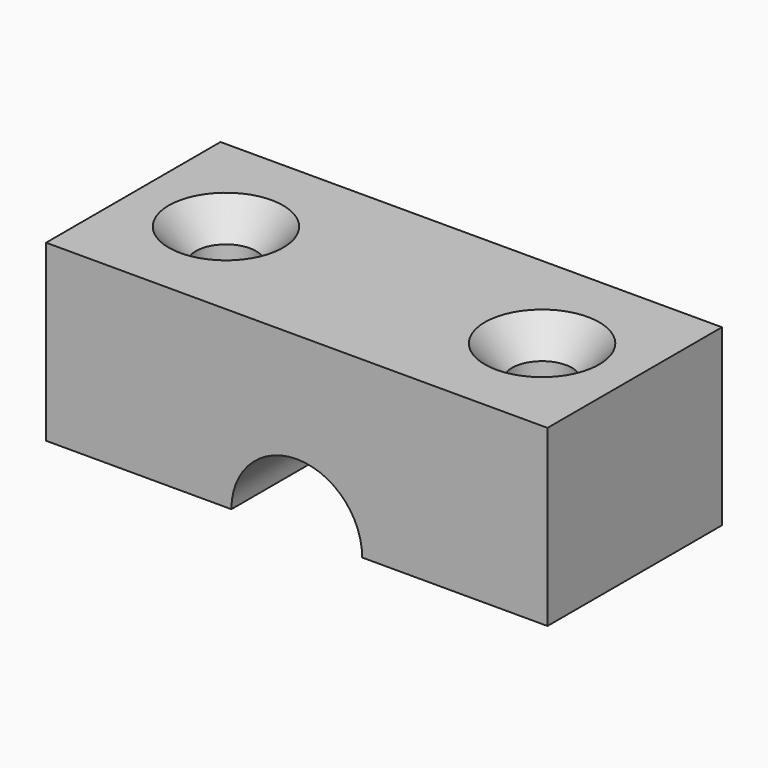
from build123d import *

# Parameters (mm, degrees)
F1_DEPTH       = 25.4
F2_D           = 8.7376
F2_DEPTH       = 29.6333418
F2_CSINK_D     = 16.6624
F2_CSINK_ANGLE = 82
F2_TIP         = 2.6250398724
F4_D           = 19.05


# Not quite as in the source:
# - a feature names something its author has since deleted; it is built from what else it names


with BuildPart() as f1:
    # F0 (on Top) → F1 (new body)
    with BuildSketch(Plane.XY):
        Polygon((36.5125, -15.875), (36.5125, 15.875), (0, 15.875), (-36.5125, 15.875), (-36.5125, -15.875), align=None)
    extrude(amount=-F1_DEPTH)

    # F2
    with Locations(Plane.XY):
        with Locations((-23.01875, 0), (23.01875, 0)):
            CounterSinkHole(F2_D / 2, F2_CSINK_D / 2, depth=F2_DEPTH, counter_sink_angle=F2_CSINK_ANGLE)
            with Locations((0, 0, -(F2_DEPTH + F2_TIP / 2))):  # 118° drill point
                Cone(0, F2_D / 2, F2_TIP, mode=Mode.SUBTRACT)

    # F4 (through all)
    with Locations(Plane.XZ.offset(15.875)):
        with Locations((0, -25.4)):
            Hole(F4_D / 2)


solid = f1.part
